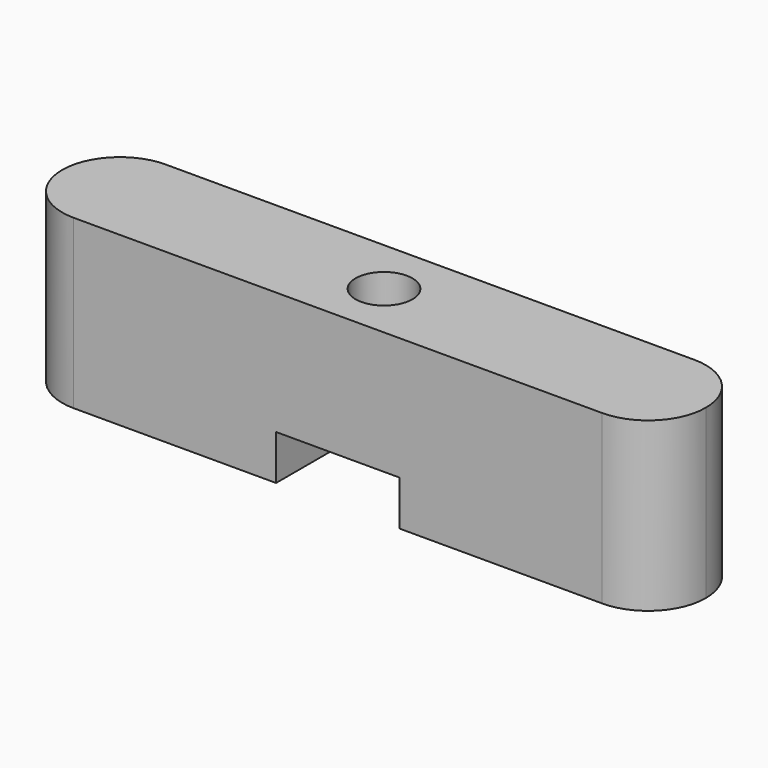
from build123d import *

# Parameters (mm, degrees)
F1_W     = 43
F1_H     = 7.7
F1_R     = 1.9
F3_DEPTH = 11.2
F2_R     = 3.4
F2_R_2   = 1.9
F4_DEPTH = 3
F5_R     = 3.84999
F6_W     = 8.2597071305
F6_H     = 7.7
F6_H_2   = 7.1181999311
F7_DEPTH = 3


# Not quite as in the source:
# - a fillet or chamfer is up to 0.001 mm smaller than in the source, because OpenCascade refuses the exact size


with BuildPart() as f3:
    # F1 (on face) → F3 (new body)
    with BuildSketch(Plane.XY):
        Rectangle(F1_W, F1_H)
        Circle(F1_R, mode=Mode.SUBTRACT)
    extrude(amount=F3_DEPTH)

    # F2 (on face) → F4 (cut)
    with BuildSketch(Plane.XY):
        Circle(F2_R)
        Circle(F2_R_2, mode=Mode.SUBTRACT)
    extrude(amount=F4_DEPTH, mode=Mode.SUBTRACT)

    # F5 (radius 3.85 in the source; OpenCascade refuses exactly that, so slightly less here)
    f5_edges = [f3.edges().sort_by_distance(p)[0] for p in [
        (-21.5, -3.85, 5.6),
        (-21.5, 3.85, 5.6),
        (21.5, -3.85, 5.6),
        (21.5, 3.85, 5.6),
    ]]
    fillet(f5_edges, radius=F5_R)

    # F6 (on face) → F7 (cut)
    with BuildSketch(Plane.XY):
        Rectangle(F6_W, F6_H)
        with Locations((0, -7.4090999655)):
            Rectangle(F6_W, F6_H_2)
        with Locations((0, 7.4090999655)):
            Rectangle(F6_W, F6_H_2)
    extrude(amount=F7_DEPTH, mode=Mode.SUBTRACT)


solid = f3.part
